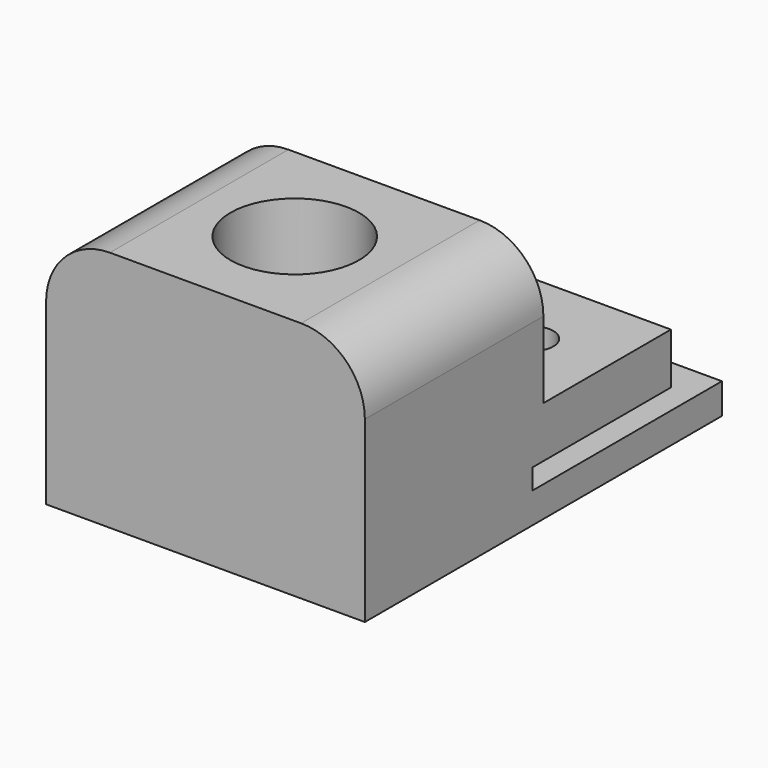
from build123d import *

# Parameters (mm, degrees)
F0_W      = 25
F0_H      = 35
F1_DEPTH  = 4
F2_W      = 25
F2_H      = 25
F2_H_2    = 5
F3_DEPTH  = 15
F4_R      = 5
F5_W      = 15
F5_H      = 12.5
F6_DEPTH  = 11
F9_D      = 3.3
F11_DEPTH = 5.5
F7_W      = 20
F7_H      = 1.6
F12_DEPTH = 25
F14_D     = 10.0838


# Not quite as in the source:
# - a feature names something its author has since deleted; it is built from what else it names


with BuildPart() as f1:
    # F0 (on Top) → F1 (new body)
    with BuildSketch(Plane.XY):
        Rectangle(F0_W, F0_H)
    extrude(amount=F1_DEPTH)

    # F2 (on face) → F3 (join)
    with BuildSketch(Plane.XY.offset(4)):
        Rectangle(F2_W, F2_H)
        with Locations((0, -15)):
            Rectangle(F2_W, F2_H_2)
    extrude(amount=F3_DEPTH)

    # F4
    f4_edges = [f1.edges().sort_by_distance(p)[0] for p in [
        (-12.5, -2.5, 19),
        (12.5, -2.5, 19),
    ]]
    fillet(f4_edges, radius=F4_R)

    # F5 (on face) → F6 (cut)
    with BuildSketch(Plane.XY.offset(19)):
        Polygon((-16.3788758218, 17.6315885037), (-16.3788758218, 0), (-7.5, 0), (-7.5, 12.5), (7.5, 12.5), (7.5, 0), (18.287928775, 0), (18.287928775, 17.6315885037), align=None)
        with Locations((0, 6.25)):
            Rectangle(F5_W, F5_H)
    extrude(amount=-F6_DEPTH, mode=Mode.SUBTRACT)

    # F9 (through all)
    with Locations(Plane.XY.offset(8)):
        with Locations((6.6282246262, 6.25), (-6.6282246262, 6.25)):
            Hole(F9_D / 2)

    # F10 (on face) → F11 (cut)
    with BuildSketch(Plane.XY):
        Polygon((-5.0405113859, 3.5), (-3.4527981456, 6.25), (-5.0405113859, 9), (-8.2159378665, 9), (-9.8036511067, 6.25), (-8.2159378665, 3.5), align=None)
        Polygon((5.0405113859, 9), (3.4527981456, 6.25), (5.0405113859, 3.5), (8.2159378665, 3.5), (9.8036511067, 6.25), (8.2159378665, 9), align=None)
    extrude(amount=F11_DEPTH, mode=Mode.SUBTRACT)

    # F7 (on face) → F12 (cut)
    with BuildSketch(Plane.YZ.offset(12.5)):
        with Locations((8.9099199928, 3.2)):
            Rectangle(F7_W, F7_H)
    extrude(amount=-F12_DEPTH, mode=Mode.SUBTRACT)

    # F14 (through all)
    with Locations(Plane.XY.offset(19)):
        with Locations((0, -8.75)):
            Hole(F14_D / 2)


solid = f1.part
